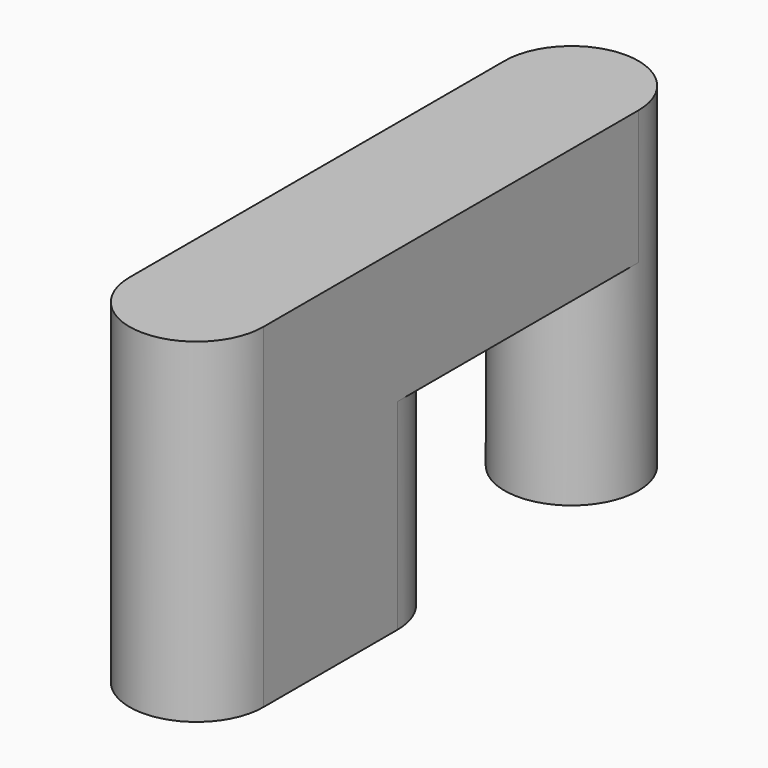
from build123d import *

# Parameters (mm, degrees)
F0_R     = 10
F1_DEPTH = 50
F3_DEPTH = 20
F5_DEPTH = 50
F6_R     = 9.99999


# Not quite as in the source:
# - a fillet or chamfer is up to 0.001 mm smaller than in the source, because OpenCascade refuses the exact size


with BuildPart() as f1:
    # F0 (on Top) → F1 (new body)
    with BuildSketch(Plane.XY):
        Circle(F0_R)
    extrude(amount=F1_DEPTH)

    # F2 (on face) → F3 (join)
    with BuildSketch(Plane.XY.offset(50)):
        with BuildLine():
            ThreePointArc((10, 0), (0, -10), (-10, 0))
            Line((-10, 0), (-10, -70))
            Line((-10, -70), (10, -70))
            Line((10, -70), (10, 0))
        make_face()
    extrude(amount=-F3_DEPTH)

    # F4 (on face) → F5 (join)
    with BuildSketch(Plane.XY.offset(50)):
        with BuildLine():
            Line((-10, -35), (-10, -70))
            ThreePointArc((-10, -70), (0, -60), (10, -70))
            Line((10, -70), (10, -35))
            Line((10, -35), (-10, -35))
        make_face()
        with BuildLine():
            ThreePointArc((10, -70), (0, -60), (-10, -70))
            Line((-10, -70), (10, -70))
        make_face()
        with BuildLine():
            Line((10, -70), (-10, -70))
            ThreePointArc((-10, -70), (0, -80), (10, -70))
        make_face()
    extrude(amount=-F5_DEPTH)

    # F6 (radius 10 in the source; OpenCascade refuses exactly that, so slightly less here)
    f6_edges = [f1.edges().sort_by_distance(p)[0] for p in [
        (10, -35, 15),
        (-10, -35, 15),
    ]]
    fillet(f6_edges, radius=F6_R)


solid = f1.part
